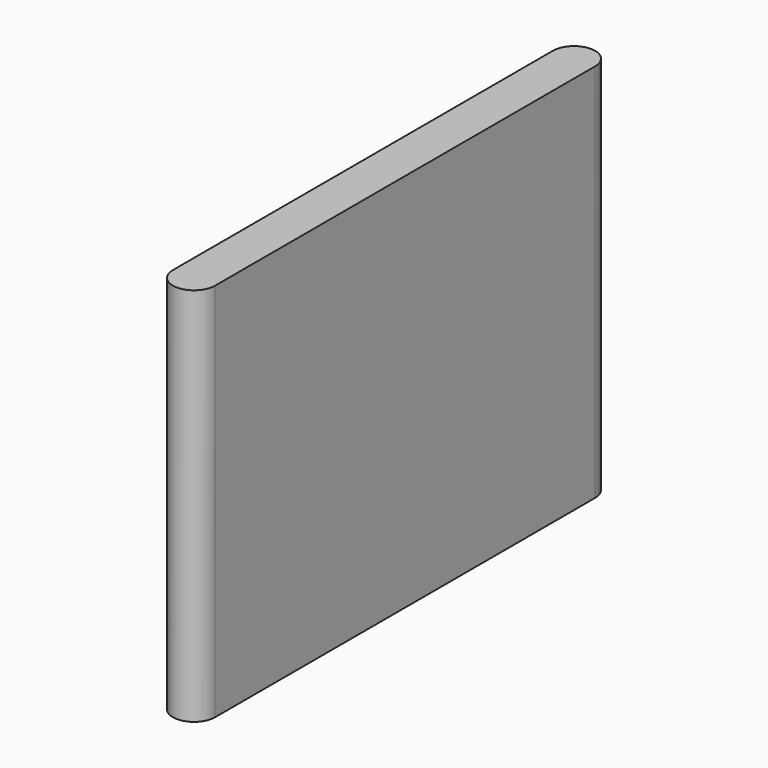
from build123d import *

# Parameters (mm, degrees)
F1_DEPTH = 18


# Not quite as in the source:
# - ends of sketch curves that miss each other by under 0.0002 mm in the source are joined


with BuildPart() as f1:
    # F0 (on Top) → F1 (new body, symmetric)
    with BuildSketch(Plane.XY):
        with BuildLine():
            Line((1.9999976953, -22.5999992664), (1.9999976953, 22.4000007336))
            ThreePointArc((1.9999976953, 22.4000007336), (2.3047e-06, 24.3999961241), (-1.9999930858, 22.4000007336))
            Line((-1.9999930858, 22.4000007336), (-1.9999976953, -22.5999992664))
            ThreePointArc((-1.9999976953, -22.5999992664), (-2.3047e-06, -24.5999992664), (1.9999976953, -22.5999992664))
        make_face()
    extrude(amount=F1_DEPTH, both=True)


solid = f1.part
